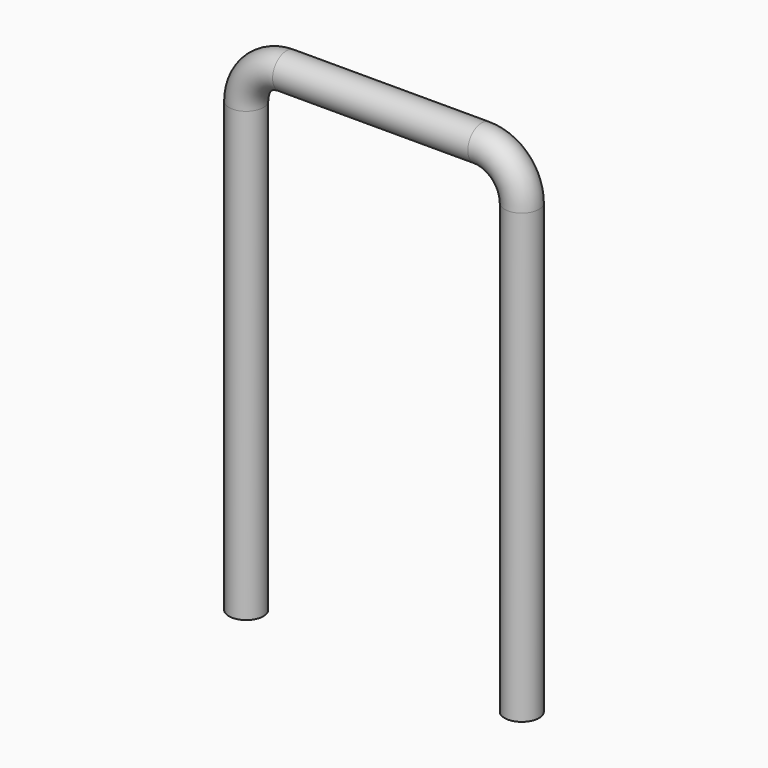
from build123d import *

# Parameters (mm, degrees)
F1_R = 3


with BuildPart() as f2:
    # F2: sweep along a path in F0
    with BuildLine(Plane.XZ) as f2_path:
        Line((-21, 0), (-21, 78))
        ThreePointArc((-21, 78), (-19.8284271247, 80.8284271247), (-17, 82))
        Line((-17, 82), (17, 82))
        ThreePointArc((17, 82), (19.8284271247, 80.8284271247), (21, 78))
        Line((21, 78), (21, 0))
    # F1 (on Top) → F2 (sweep)
    with BuildSketch(Plane.XY):
        with Locations((-24, 0)):
            Circle(F1_R)
    sweep(path=f2_path.line)


solid = f2.part
